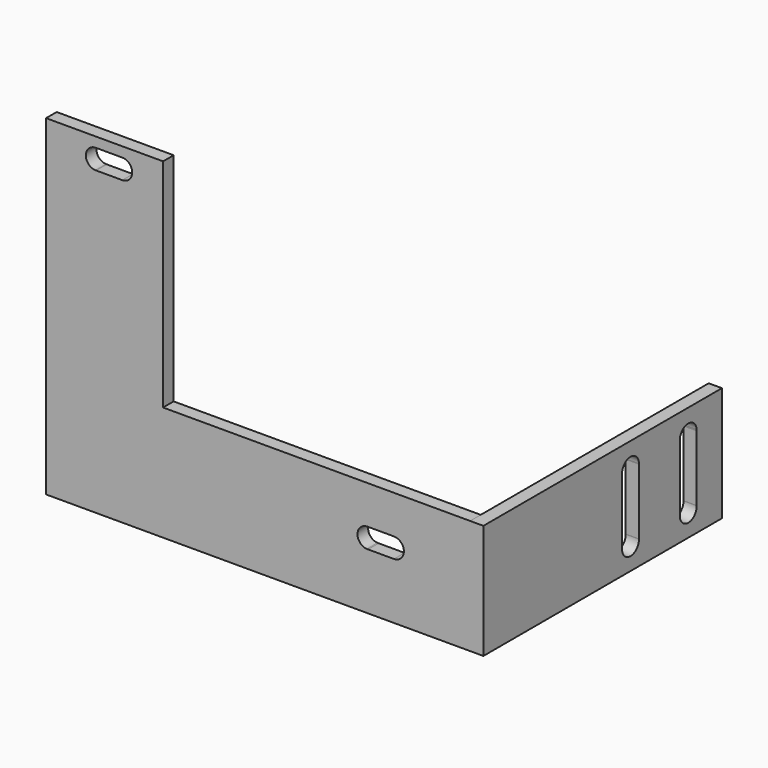
from build123d import *

# Parameters (mm, degrees)
F1_DEPTH = 1
F2_W     = 45
F2_H     = 17.293657
F3_DEPTH = 1


# Not quite as in the source:
# - ends of sketch curves that miss each other by under 0.0002 mm in the source are joined


with BuildPart() as f1:
    # F0 (on Front) → F1 (new body, symmetric)
    with BuildSketch(Plane.XZ):
        Polygon((-32.5, -25), (32.5, -25), (32.5, -7.706343), (-14.84501, -7.706343), (-14.84501, 25), (-32.5, 25), align=None)
        with BuildLine():
            ThreePointArc((15.901332, -16.496751), (14.500453, -14.963122), (15.975024, -13.500208))
            Line((15.975024, -13.500208), (19.999923, -13.5))
            ThreePointArc((19.999923, -13.5), (21.060633, -13.939312), (21.5, -15))
            ThreePointArc((21.5, -15), (21.06024, -16.06108), (19.998811, -16.5))
            Line((19.998811, -16.5), (16.096295, -16.496906))
            ThreePointArc((16.096295, -16.496906), (15.998811, -16.5), (15.901332, -16.496751))
        make_face(mode=Mode.SUBTRACT)
        with BuildLine():
            ThreePointArc((-25.061961, 20.50128), (-26.499497, 22.038851), (-24.984268, 23.499918))
            Line((-24.984268, 23.499918), (-21.000031, 23.5))
            ThreePointArc((-21.000031, 23.5), (-19.939351, 23.060671), (-19.5, 22))
            ThreePointArc((-19.5, 22), (-19.939507, 20.939173), (-21.000473, 20.5))
            Line((-21.000473, 20.5), (-24.938984, 20.501241))
            ThreePointArc((-24.938984, 20.501241), (-25.000473, 20.5), (-25.061961, 20.50128))
        make_face(mode=Mode.SUBTRACT)
    extrude(amount=F1_DEPTH, both=True)

    # F2 (on face) → F3 (join, symmetric)
    with BuildSketch(Plane.YZ.offset(32.5)):
        with Locations((21.5, -16.353171)):
            Rectangle(F2_W, F2_H)
        with BuildLine():
            ThreePointArc((28.349491, -21.374032), (28.349873, -21.394217), (28.35, -21.414405))
            ThreePointArc((28.35, -21.414405), (26.729813, -23.014278), (25.150509, -21.374034))
            Line((25.150509, -21.374034), (25.150429, -11.451472))
            ThreePointArc((25.150429, -11.451472), (25.15, -11.414405), (25.150429, -11.377338))
            ThreePointArc((25.150429, -11.377338), (26.749999, -9.814405), (28.349571, -11.377336))
            ThreePointArc((28.349571, -11.377336), (28.349893, -11.395869), (28.35, -11.414405))
            ThreePointArc((28.35, -11.414405), (28.349873, -11.434593), (28.349491, -11.454778))
            Line((28.349491, -11.454778), (28.349491, -21.374032))
        make_face(mode=Mode.SUBTRACT)
        with BuildLine():
            ThreePointArc((39.249491, -21.374032), (39.249873, -21.394217), (39.25, -21.414405))
            ThreePointArc((39.25, -21.414405), (37.585541, -23.013106), (36.055194, -21.285591))
            Line((36.055194, -21.285591), (36.055194, -11.543219))
            ThreePointArc((36.055194, -11.543219), (36.05, -11.414405), (36.055194, -11.285591))
            ThreePointArc((36.055194, -11.285591), (37.65, -9.814405), (39.244806, -11.285591))
            Line((39.244806, -11.285591), (39.249491, -11.285591))
            Line((39.249491, -11.285591), (39.249491, -11.374032))
            ThreePointArc((39.249491, -11.374032), (39.249873, -11.394217), (39.25, -11.414405))
            ThreePointArc((39.25, -11.414405), (39.249873, -11.434593), (39.249491, -11.454778))
            Line((39.249491, -11.454778), (39.249491, -21.374032))
        make_face(mode=Mode.SUBTRACT)
    extrude(amount=F3_DEPTH, both=True)


solid = f1.part
